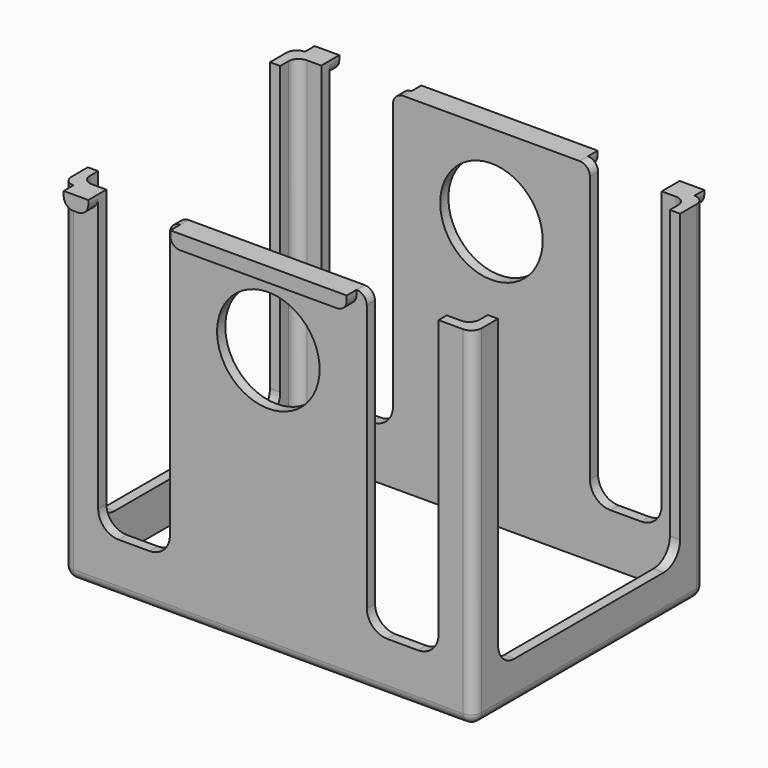
from build123d import *

# Parameters (mm, degrees)
F1_DEPTH  = 170
F2_R      = 25
F3_DEPTH  = 250
F5_DEPTH  = 210
F6_R      = 5
F8_DEPTH  = 6
F9_R      = 4.99999
F11_DEPTH = 6


# Not quite as in the source:
# - a fillet or chamfer is up to 0.001 mm smaller than in the source, because OpenCascade refuses the exact size


with BuildPart() as f1:
    # F0 (on Top) → F1 (new body)
    with BuildSketch(Plane.XY):
        with BuildLine():
            ThreePointArc((100, 65.5), (98.5355339059, 69.0355339059), (95, 70.5))
            Line((95, 70.5), (-95, 70.5))
            ThreePointArc((-95, 70.5), (-98.5355339059, 69.0355339059), (-100, 65.5))
            Line((-100, 65.5), (-100, -65.5))
            ThreePointArc((-100, -65.5), (-98.5355339059, -69.0355339059), (-95, -70.5))
            Line((-95, -70.5), (95, -70.5))
            ThreePointArc((95, -70.5), (98.5355339059, -69.0355339059), (100, -65.5))
            Line((100, -65.5), (100, 65.5))
        make_face()
        with BuildLine():
            Line((-90, 65.5), (90, 65.5))
            ThreePointArc((90, 65.5), (93.5355339059, 64.0355339059), (95, 60.5))
            Line((95, 60.5), (95, -60.5))
            ThreePointArc((95, -60.5), (93.5355339059, -64.0355339059), (90, -65.5))
            Line((90, -65.5), (-90, -65.5))
            ThreePointArc((-90, -65.5), (-93.5355339059, -64.0355339059), (-95, -60.5))
            Line((-95, -60.5), (-95, 60.5))
            ThreePointArc((-95, 60.5), (-93.5355339059, 64.0355339059), (-90, 65.5))
        make_face(mode=Mode.SUBTRACT)
    extrude(amount=F1_DEPTH)

    # F2 (on face) → F3 (cut)
    with BuildSketch(Plane.XZ.offset(70.5)):
        with Locations((0, 130)):
            Circle(F2_R)
        with BuildLine():
            Line((-48, 170), (-83, 170))
            Line((-83, 170), (-83, 35))
            ThreePointArc((-83, 35), (-80.0710678119, 27.9289321881), (-73, 25))
            Line((-73, 25), (-58, 25))
            ThreePointArc((-58, 25), (-50.9289321881, 27.9289321881), (-48, 35))
            Line((-48, 35), (-48, 170))
        make_face()
        with BuildLine():
            Line((83, 170), (48, 170))
            Line((48, 170), (48, 35))
            ThreePointArc((48, 35), (50.9289321881, 27.9289321881), (58, 25))
            Line((58, 25), (73, 25))
            ThreePointArc((73, 25), (80.0710678119, 27.9289321881), (83, 35))
            Line((83, 35), (83, 170))
        make_face()
    extrude(amount=-F3_DEPTH, mode=Mode.SUBTRACT)

    # F4 (on face) → F5 (cut)
    with BuildSketch(Plane.YZ.offset(100)):
        with BuildLine():
            Line((55.5, 170), (-55.5, 170))
            Line((-55.5, 170), (-55.5, 30))
            ThreePointArc((-55.5, 30), (-52.5710678119, 22.9289321881), (-45.5, 20))
            Line((-45.5, 20), (45.5, 20))
            ThreePointArc((45.5, 20), (52.5710678119, 22.9289321881), (55.5, 30))
            Line((55.5, 30), (55.5, 170))
        make_face()
    extrude(amount=-F5_DEPTH, mode=Mode.SUBTRACT)

    # F6
    f6_edges = [f1.edges().sort_by_distance(p)[0] for p in [
        (-48, -68, 170),
        (48, -68, 170),
        (48, 68, 170),
        (-48, 68, 170),
    ]]
    fillet(f6_edges, radius=F6_R)

    # F7 (on face) → F8 (join)
    with BuildSketch(Plane.XZ.offset(70.5)):
        with BuildLine():
            ThreePointArc((-88, 163), (-84.4644660941, 164.4644660941), (-83, 168))
            Line((-83, 168), (-83, 170))
            Line((-83, 170), (-95, 170))
            Line((-95, 170), (-95, 167.7))
            ThreePointArc((-95, 167.7), (-93.6234018716, 164.3765981284), (-90.3, 163))
            Line((-90.3, 163), (-88, 163))
        make_face()
        with BuildLine():
            Line((43, 170), (-43, 170))
            Line((-43, 170), (-43, 167.7))
            ThreePointArc((-43, 167.7), (-41.6234018716, 164.3765981284), (-38.3, 163))
            Line((-38.3, 163), (38.3, 163))
            ThreePointArc((38.3, 163), (41.6234018716, 164.3765981284), (43, 167.7))
            Line((43, 167.7), (43, 170))
        make_face()
    extrude(amount=F8_DEPTH)

    # F9 (radius 5 in the source; OpenCascade refuses exactly that, so slightly less here)
    f9_edges = [f1.edges().sort_by_distance(p)[0] for p in [
        (-100, 0, 0),
    ]]
    fillet(f9_edges, radius=F9_R)

    # F10 (on face) → F11 (join)
    with BuildSketch(Plane(origin=(0, 70.5, 0), x_dir=(-1, 0, 0), z_dir=(0, 1, 0))):
        with BuildLine():
            ThreePointArc((-88, 163), (-84.4644660941, 164.4644660941), (-83, 168))
            Line((-83, 168), (-83, 170))
            Line((-83, 170), (-95, 170))
            Line((-95, 170), (-95, 168))
            ThreePointArc((-95, 168), (-93.5355339059, 164.4644660941), (-90, 163))
            Line((-90, 163), (-88, 163))
        make_face()
        with BuildLine():
            Line((43, 170), (-43, 170))
            Line((-43, 170), (-43, 168))
            ThreePointArc((-43, 168), (-41.5355339059, 164.4644660941), (-38, 163))
            Line((-38, 163), (38, 163))
            ThreePointArc((38, 163), (41.5355339059, 164.4644660941), (43, 168))
            Line((43, 168), (43, 170))
        make_face()
        with BuildLine():
            Line((83, 170), (83, 168))
            ThreePointArc((83, 168), (84.4644660941, 164.4644660941), (88, 163))
            Line((88, 163), (90, 163))
            ThreePointArc((90, 163), (93.5355339059, 164.4644660941), (95, 168))
            Line((95, 168), (95, 170))
            Line((95, 170), (83, 170))
        make_face()
    extrude(amount=F11_DEPTH)


solid = f1.part
